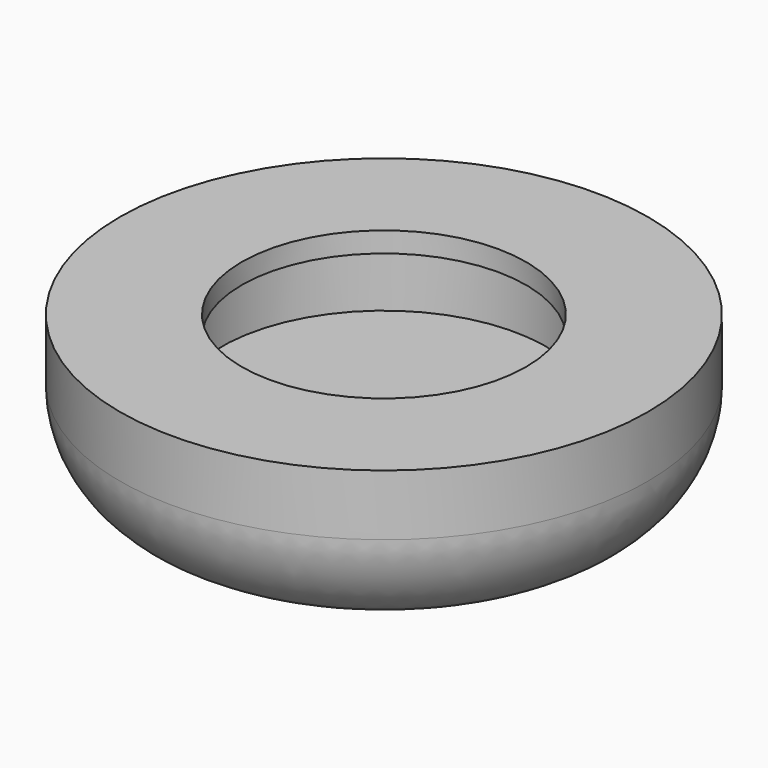
from build123d import *

# Parameters (mm, degrees)
F0_R        = 13
F0_R_2      = 1.2126826201
F0_R_3      = 8
F0_R_4      = 7
F1_DEPTH    = 2
F2_DEPTH    = 6
F4_R        = 13
F4_R_2      = 8
F4_R_3      = 7
F5_DEPTH    = 1
F2_FACE_R   = 13
F2_FACE_R_2 = 1.2126826201
F6_DEPTH    = 1
F7_DEPTH    = 2
F8_R        = 4.999


# Not quite as in the source:
# - a fillet or chamfer is up to 0.001 mm smaller than in the source, because OpenCascade refuses the exact size


with BuildPart() as f1:
    # F0 (on Top) → F1 (new body)
    with BuildSketch(Plane.XY):
        Circle(F0_R)
        with Locations((0, -10.5861881748)):
            Circle(F0_R_2, mode=Mode.SUBTRACT)
        Circle(F0_R_3, mode=Mode.SUBTRACT)
        Circle(F0_R_3)
        Circle(F0_R_4, mode=Mode.SUBTRACT)
        Circle(F0_R_4)
    extrude(amount=F1_DEPTH)

    # F0 (on Top) → F2 (join)
    with BuildSketch(Plane.XY):
        Circle(F0_R)
        with Locations((0, -10.5861881748)):
            Circle(F0_R_2, mode=Mode.SUBTRACT)
        Circle(F0_R_3, mode=Mode.SUBTRACT)
    extrude(amount=F2_DEPTH)

    # F4 (on offset) → F5 (join)
    with BuildSketch(Plane.XY.offset(6)):
        Circle(F4_R)
        Circle(F4_R_2, mode=Mode.SUBTRACT)
        Circle(F4_R_2)
        Circle(F4_R_3, mode=Mode.SUBTRACT)
    extrude(amount=-F5_DEPTH)

    # F2_face (on face) + F0 (on Top) → F6 (join)
    with BuildSketch(Plane(origin=(0, 0.0929272063, 0), x_dir=(1, 0, 0), z_dir=(0, 0, -1))):
        with Locations((0, 0.0929272063)):
            Circle(F2_FACE_R)
        with Locations((0, 10.6791153811)):
            Circle(F2_FACE_R_2, mode=Mode.SUBTRACT)
    with BuildSketch(Plane.XY):
        Circle(F0_R_4)
    extrude(amount=-F6_DEPTH, dir=(0, 0, -1))

    # F0 (on Top) → F7 (join)
    with BuildSketch(Plane.XY):
        Circle(F0_R)
        with Locations((0, -10.5861881748)):
            Circle(F0_R_2, mode=Mode.SUBTRACT)
        Circle(F0_R_3, mode=Mode.SUBTRACT)
    extrude(amount=-F7_DEPTH)

    # F8 (radius 5 in the source; OpenCascade refuses exactly that, so slightly less here)
    f8_edges = [f1.edges().sort_by_distance(p)[0] for p in [
        (-13, 0, -2),
    ]]
    fillet(f8_edges, radius=F8_R)


solid = f1.part
